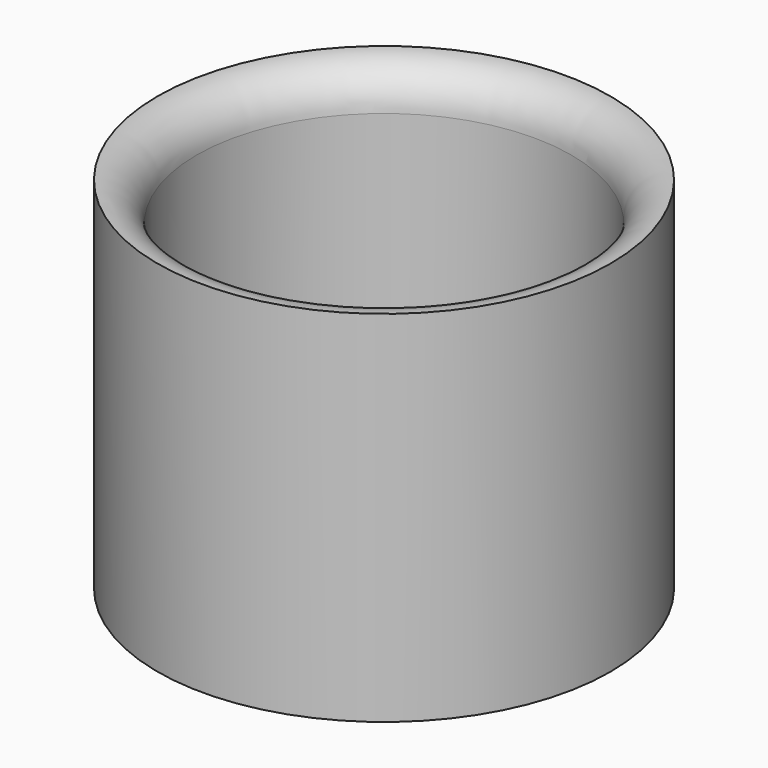
from build123d import *

# Parameters (mm, degrees)
F0_R     = 14.5
F0_R_2   = 12
F1_DEPTH = 23
F2_R     = 2.49999


# Not quite as in the source:
# - a fillet or chamfer is up to 0.001 mm smaller than in the source, because OpenCascade refuses the exact size


with BuildPart() as f1:
    # F0 (on Top) → F1 (new body)
    with BuildSketch(Plane.XY):
        Circle(F0_R)
        Circle(F0_R_2, mode=Mode.SUBTRACT)
    extrude(amount=F1_DEPTH)

    # F2 (radius 2.5 in the source; OpenCascade refuses exactly that, so slightly less here)
    f2_edges = [f1.edges().sort_by_distance(p)[0] for p in [
        (-12, 0, 23),
    ]]
    fillet(f2_edges, radius=F2_R)


solid = f1.part
